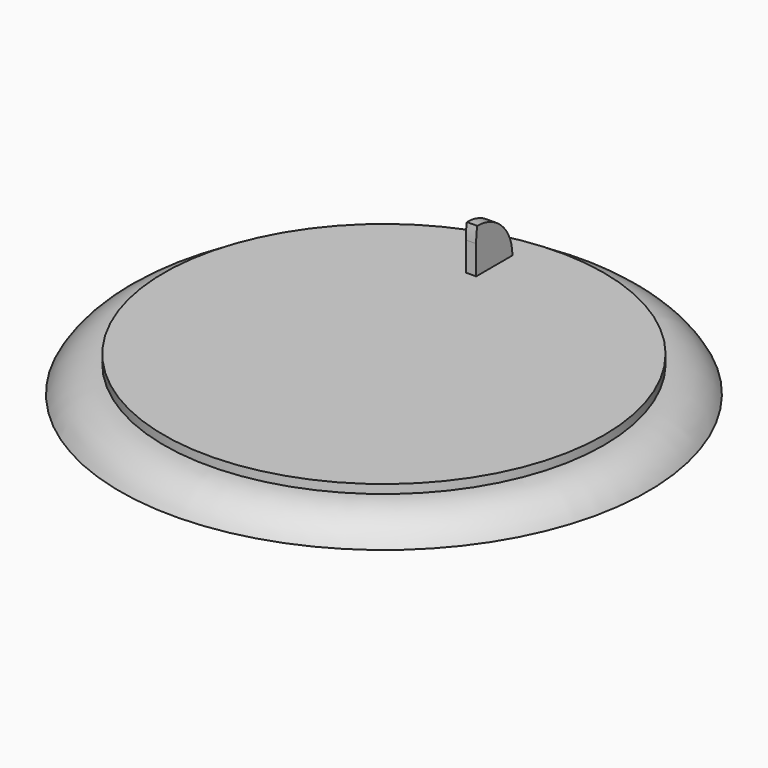
from build123d import *

# Parameters (mm, degrees)
F3_R        = 25
F4_DEPTH    = 1
F5_W        = 1.1802830268
F5_H        = 5.150327459
F6_DEPTH    = 5
F7_R        = 4.99999
F8_T1_DEPTH = 9.8176261194


# Not quite as in the source:
# - a fillet or chamfer that OpenCascade refuses, or shapes differently, is made with other operations: its cross-section is extruded or revolved along the edge and cut away or added
# - a fillet or chamfer is up to 0.001 mm smaller than in the source, because OpenCascade refuses the exact size


with BuildPart() as f1:
    # F0 (on Front) → F1 (revolve)
    with BuildSketch(Plane.XZ):
        with BuildLine():
            Line((-30, 0), (0, 0))
            Line((0, 0), (0, 3))
            Line((0, 3), (-25, 3))
            ThreePointArc((-25, 3), (-27.9154759474, 2.1924599124), (-30, 0))
        make_face()
    revolve(axis=Axis((0, 0, 1.5), (0, 0, 1)))

    # F3 (on face) → F4 (join)
    with BuildSketch(Plane.XY.offset(3)):
        Circle(F3_R)
    extrude(amount=F4_DEPTH)

    # F5 (on face) → F6 (join)
    with BuildSketch(Plane.XY.offset(4)):
        with Locations((-3.5133393249, 19.3324619904)):
            Rectangle(F5_W, F5_H)
    extrude(amount=F6_DEPTH)

    # F7 (radius 5 in the source; OpenCascade refuses exactly that, so slightly less here)
    f7_edges = [f1.edges().sort_by_distance(p)[0] for p in [
        (-3.513339, 21.907626, 9),
    ]]
    fillet(f7_edges, radius=F7_R)

    # F8: fillet of radius 10 on 1 edges, made by hand

    # F8_s2 → F8_t1 (cut)
    with BuildSketch(Plane.YZ.offset(-8.4221523845)):
        with BuildLine():
            ThreePointArc((16.9076357199, 9), (16.7949535216, 8.1395303981), (16.7572982609, 7.2725313815))
            Line((16.7572982609, 7.2725313815), (16.7572982609, 9))
            Line((16.7572982609, 9), (16.9076357199, 9))
        make_face()
    extrude(amount=F8_T1_DEPTH, mode=Mode.SUBTRACT)


solid = f1.part
